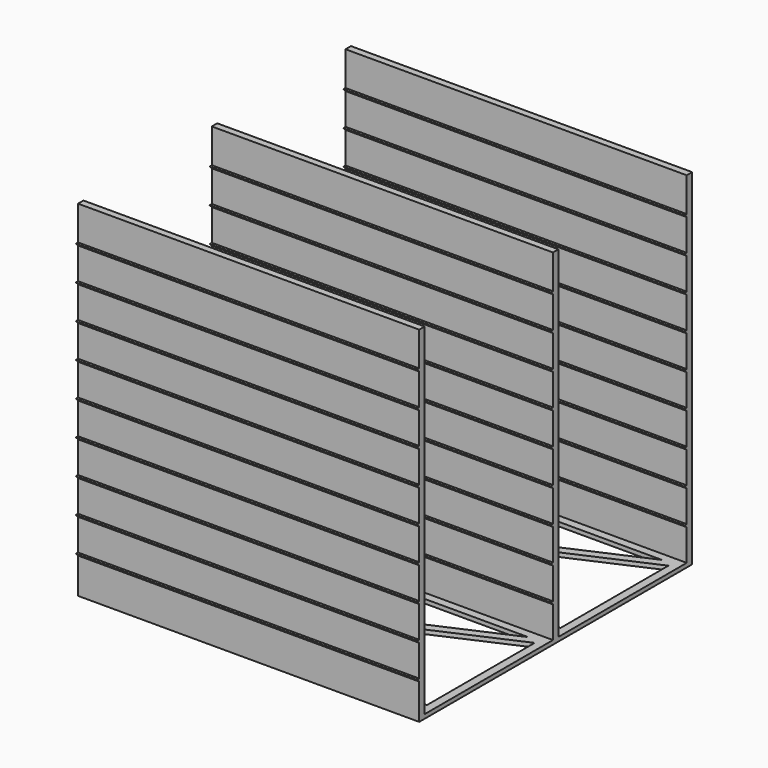
from build123d import *

# Parameters (mm, degrees)
F0_W     = 50
F0_H     = 23.5
F0_H_2   = 1
F1_DEPTH = 0.6
F2_DEPTH = 50
F4_DEPTH = 50


# Not quite as in the source:
# - a feature names something its author has since deleted; it is built from what else it names


with BuildPart() as f1:
    # F0 (on Top) → F1 (new body)
    with BuildSketch(Plane.XY):
        with Locations((0, 12.25)):
            Rectangle(F0_W, F0_H)
        Polygon((-23.8, 22.1436935786), (-23.8, 22.8), (-22.3194224806, 22.8), (22.3194224806, 22.8), (23.8, 22.8), (23.8, 22.1436935786), (23.8, 2.3563064214), (23.8, 1.7), (22.3194224806, 1.7), (-22.3194224806, 1.7), (-23.8, 1.7), (-23.8, 2.3563064214), align=None, mode=Mode.SUBTRACT)
        with Locations((0, -12.25)):
            Rectangle(F0_W, F0_H)
        Polygon((-22.3194224806, -22.8), (-23.8, -22.8), (-23.8, -22.1436935786), (-23.8, -2.3563064214), (-23.8, -1.7), (-22.3194224806, -1.7), (22.3194224806, -1.7), (23.8, -1.7), (23.8, -2.3563064214), (23.8, -22.1436935786), (23.8, -22.8), (22.3194224806, -22.8), align=None, mode=Mode.SUBTRACT)
        with Locations((0, -24.5)):
            Rectangle(F0_W, F0_H_2)
        Rectangle(F0_W, F0_H_2)
        with Locations((0, 24.5)):
            Rectangle(F0_W, F0_H_2)
        Polygon((-22.3194224806, 22.8), (-23.8, 22.8), (-23.8, 22.1436935786), (-1.4805775194, 12.25), (0, 12.9063064214), align=None)
        Polygon((23.8, 22.8), (22.3194224806, 22.8), (0, 12.9063064214), (1.4805775194, 12.25), (23.8, 22.1436935786), align=None)
        Polygon((1.4805775194, 12.25), (0, 12.9063064214), (-1.4805775194, 12.25), (0, 11.5936935786), align=None)
        Polygon((23.8, 2.3563064214), (1.4805775194, 12.25), (0, 11.5936935786), (22.3194224806, 1.7), (23.8, 1.7), align=None)
        Polygon((-1.4805775194, 12.25), (-23.8, 2.3563064214), (-23.8, 1.7), (-22.3194224806, 1.7), (0, 11.5936935786), align=None)
        Polygon((-23.8, -1.7), (-23.8, -2.3563064214), (-1.4805775194, -12.25), (0, -11.5936935786), (-22.3194224806, -1.7), align=None)
        Polygon((0, -11.5936935786), (-1.4805775194, -12.25), (0, -12.9063064214), (1.4805775194, -12.25), align=None)
        Polygon((22.3194224806, -1.7), (0, -11.5936935786), (1.4805775194, -12.25), (23.8, -2.3563064214), (23.8, -1.7), align=None)
        Polygon((0, -12.9063064214), (22.3194224806, -22.8), (23.8, -22.8), (23.8, -22.1436935786), (1.4805775194, -12.25), align=None)
        Polygon((-23.8, -22.1436935786), (-23.8, -22.8), (-22.3194224806, -22.8), (0, -12.9063064214), (-1.4805775194, -12.25), align=None)
    extrude(amount=-F1_DEPTH)

    # F0 (on Top) → F2 (join)
    with BuildSketch(Plane.XY):
        with Locations((0, 24.5)):
            Rectangle(F0_W, F0_H_2)
        Rectangle(F0_W, F0_H_2)
        with Locations((0, -24.5)):
            Rectangle(F0_W, F0_H_2)
    extrude(amount=F2_DEPTH)

    # F3 (on face) → F4 (join, through all)
    with BuildSketch(Plane(origin=(-25, 0, 0), x_dir=(0, -1, 0), z_dir=(-1, 0, 0))):
        Polygon((-24, 45), (-24, 44.6), (-23.6, 45), align=None)
        Polygon((-24, 40), (-24, 39.6), (-23.6, 40), align=None)
        Polygon((-24, 35), (-24, 34.6), (-23.6, 35), align=None)
        Polygon((-24, 30), (-24, 29.6), (-23.6, 30), align=None)
        Polygon((-24, 25), (-24, 24.6), (-23.6, 25), align=None)
        Polygon((-24, 20), (-24, 19.6), (-23.6, 20), align=None)
        Polygon((-24, 15), (-24, 14.6), (-23.6, 15), align=None)
        Polygon((-24, 10), (-24, 9.6), (-23.6, 10), align=None)
        Polygon((-24, 5), (-24, 4.6), (-23.6, 5), align=None)
        Polygon((0.9, 5), (0.5, 5), (0.5, 4.6), align=None)
        Polygon((0.9, 10), (0.5, 10), (0.5, 9.6), align=None)
        Polygon((0.9, 15), (0.5, 15), (0.5, 14.6), align=None)
        Polygon((0.9, 20), (0.5, 20), (0.5, 19.6), align=None)
        Polygon((0.9, 25), (0.5, 25), (0.5, 24.6), align=None)
        Polygon((0.9, 30), (0.5, 30), (0.5, 29.6), align=None)
        Polygon((0.9, 35), (0.5, 35), (0.5, 34.6), align=None)
        Polygon((0.9, 40), (0.5, 40), (0.5, 39.6), align=None)
        Polygon((0.9, 45), (0.5, 45), (0.5, 44.6), align=None)
        Polygon((25.4, 45), (25, 45), (25, 44.6), align=None)
        Polygon((25.4, 40), (25, 40), (25, 39.6), align=None)
        Polygon((25.4, 35), (25, 35), (25, 34.6), align=None)
        Polygon((25, 30), (25, 29.6), (25.4, 30), align=None)
        Polygon((25, 25), (25, 24.6), (25.4, 25), align=None)
        Polygon((25, 20), (25, 19.6), (25.4, 20), align=None)
        Polygon((25, 15), (25, 14.6), (25.4, 15), align=None)
        Polygon((25, 10), (25, 9.6), (25.4, 10), align=None)
        Polygon((25, 5), (25, 4.6), (25.4, 5), align=None)
    extrude(amount=-F4_DEPTH)


solid = f1.part
